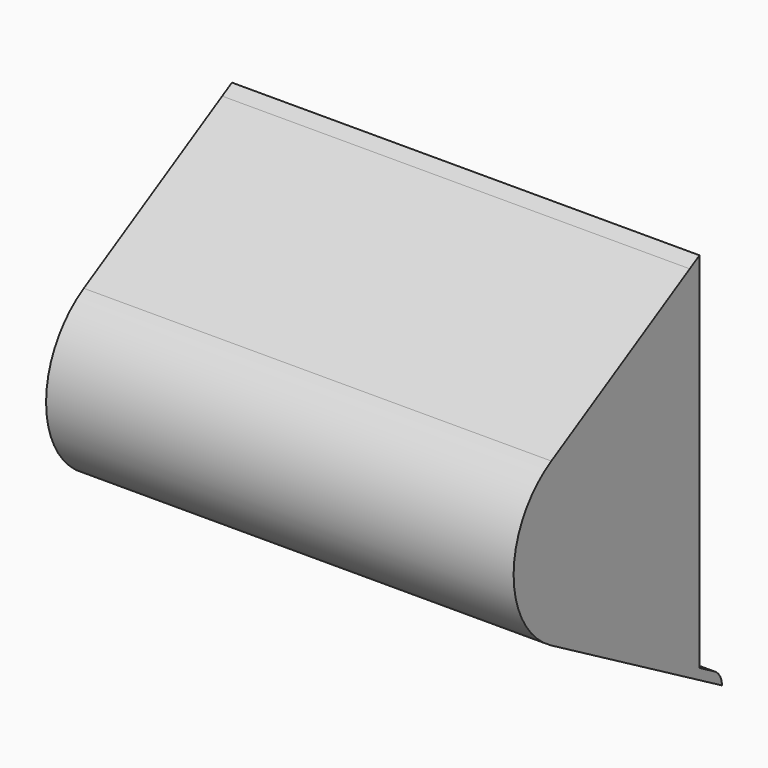
from build123d import *

# Parameters (mm, degrees)
F1_DEPTH      = 25
F1_DEPTH_BACK = 25
F2_DEPTH      = 25
F2_DEPTH_BACK = 25
F3_T1_DEPTH   = 55.8032253547
F4_START      = 24
F4_DEPTH      = 1


# Not quite as in the source:
# - a fillet or chamfer that OpenCascade refuses, or shapes differently, is made with other operations: its cross-section is extruded or revolved along the edge and cut away or added


with BuildPart() as f1:
    # F0 (on Right) → F1 (new body, two sides)
    with BuildSketch(Plane.YZ) as f1_sk:
        with BuildLine():
            ThreePointArc((-0.474586405, -1.4229433383), (-0.9510831171, -1.1599314222), (-1.3023647132, -0.7442084075))
            Line((-1.3023647132, -0.7442084075), (-19.8057450128, -11.3175685788))
            ThreePointArc((-19.8057450128, -11.3175685788), (-21.1992188281, -12.2788787263), (-22.4105694786, -13.461467444))
            ThreePointArc((-22.4105694786, -13.461467444), (-24.7010613056, -21.6868174799), (-19.8057450128, -28.6824314212))
            Line((-19.8057450128, -28.6824314212), (0, -40))
            Line((0, -40), (0, -38.8482488931))
            Line((0, -38.8482488931), (-19.3096060745, -27.8141882791))
            ThreePointArc((-19.3096060745, -27.8141882791), (-23.8443556293, -20), (-19.3096060745, -12.1858117209))
            Line((-19.3096060745, -12.1858117209), (-0.474586405, -1.4229433383))
        make_face()
        with BuildLine():
            Line((0, 0), (-1.3023647132, -0.7442084075))
            ThreePointArc((-1.3023647132, -0.7442084075), (-0.9510831171, -1.1599314222), (-0.474586405, -1.4229433383))
            Line((-0.474586405, -1.4229433383), (0, -1.1517511069))
            Line((0, -1.1517511069), (0, 0))
        make_face()
    extrude(amount=F1_DEPTH)
    extrude(f1_sk.sketch, amount=-F1_DEPTH_BACK)

    # F0 (on Right) → F2 (join, two sides)
    with BuildSketch(Plane.YZ) as f2_sk:
        Polygon((3, -40.5625346074), (0, -38.8482488931), (0, -40), (3, -41.7142857143), align=None)
    extrude(amount=F2_DEPTH)
    extrude(f2_sk.sketch, amount=-F2_DEPTH_BACK)

    # F3: fillet of radius 2 on 1 edges, made by hand

    # F3_s2 → F3_t1 (cut)
    with BuildSketch(Plane.YZ.offset(-27.9016126774)):
        with BuildLine():
            ThreePointArc((1.9922778767, -39.9866933941), (2.7298201862, -40.7193260419), (3, -41.7231796783))
            Line((3, -41.7231796783), (3, -40.5625346074))
            Line((3, -40.5625346074), (1.9922778767, -39.9866933941))
        make_face()
    extrude(amount=F3_T1_DEPTH, mode=Mode.SUBTRACT)

    # F0 (on Right) → F4 (join)
    with BuildSketch(Plane.YZ.offset(F4_START)):
        with BuildLine():
            Line((0, -38.8482488931), (0, -1.5))
            ThreePointArc((0, -1.5), (-0.2404006993, -1.4806105172), (-0.474586405, -1.4229433383))
            Line((-0.474586405, -1.4229433383), (-19.3096060745, -12.1858117209))
            ThreePointArc((-19.3096060745, -12.1858117209), (-23.8443556293, -20), (-19.3096060745, -27.8141882791))
            Line((-19.3096060745, -27.8141882791), (0, -38.8482488931))
        make_face()
        with BuildLine():
            ThreePointArc((-0.474586405, -1.4229433383), (-0.2404006993, -1.4806105172), (0, -1.5))
            Line((0, -1.5), (0, -1.1517511069))
            Line((0, -1.1517511069), (-0.474586405, -1.4229433383))
        make_face()
    extrude(amount=F4_DEPTH)


solid = f1.part
